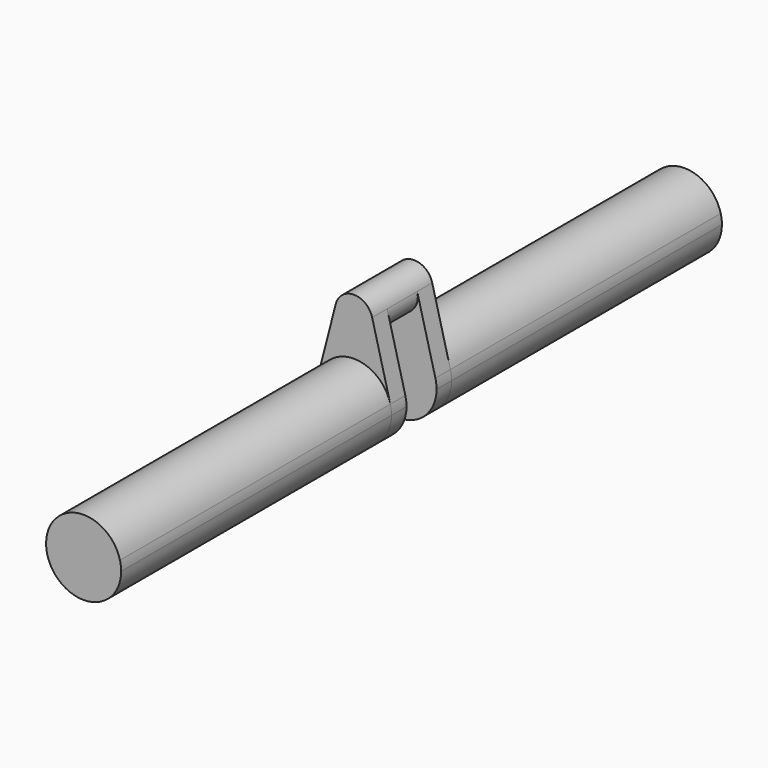
from build123d import *

# Parameters (mm, degrees)
F1_DEPTH = 5
F2_DEPTH = 50
F3_DEPTH = 2.5


with BuildPart() as f1:
    # F0 (on Front) → F1 (new body, symmetric)
    with BuildSketch(Plane.XZ):
        with BuildLine():
            ThreePointArc((2.5, 10), (2.4800742407, 10.3150107312), (2.4206145914, 10.625))
            ThreePointArc((2.4206145914, 10.625), (0, 12.5), (-2.4206145914, 10.625))
            ThreePointArc((-2.4206145914, 10.625), (-0.3150107312, 7.5199257593), (2.5, 10))
        make_face()
        with BuildLine():
            ThreePointArc((-4.8412291828, 1.25), (0, 5), (4.8412291828, 1.25))
            Line((4.8412291828, 1.25), (2.4206145914, 10.625))
            ThreePointArc((2.4206145914, 10.625), (2.4800742407, 10.3150107312), (2.5, 10))
            ThreePointArc((2.5, 10), (-0.3150107312, 7.5199257593), (-2.4206145914, 10.625))
            Line((-2.4206145914, 10.625), (-4.8412291828, 1.25))
        make_face()
        with BuildLine():
            ThreePointArc((-4.8412291828, 1.25), (-0.6300214624, -4.9601484813), (5, 0))
            ThreePointArc((5, 0), (4.9601484813, 0.6300214624), (4.8412291828, 1.25))
            ThreePointArc((4.8412291828, 1.25), (0, 5), (-4.8412291828, 1.25))
        make_face()
    extrude(amount=F1_DEPTH, both=True)

    # F0 (on Front) → F2 (join, symmetric)
    with BuildSketch(Plane.XZ):
        with BuildLine():
            ThreePointArc((-4.8412291828, 1.25), (-0.6300214624, -4.9601484813), (5, 0))
            ThreePointArc((5, 0), (4.9601484813, 0.6300214624), (4.8412291828, 1.25))
            ThreePointArc((4.8412291828, 1.25), (0, 5), (-4.8412291828, 1.25))
        make_face()
    extrude(amount=F2_DEPTH, both=True)

    # F0 (on Front) → F3 (cut, symmetric)
    with BuildSketch(Plane.XZ):
        with BuildLine():
            ThreePointArc((-4.8412291828, 1.25), (0, 5), (4.8412291828, 1.25))
            Line((4.8412291828, 1.25), (2.4206145914, 10.625))
            ThreePointArc((2.4206145914, 10.625), (2.4800742407, 10.3150107312), (2.5, 10))
            ThreePointArc((2.5, 10), (-0.3150107312, 7.5199257593), (-2.4206145914, 10.625))
            Line((-2.4206145914, 10.625), (-4.8412291828, 1.25))
        make_face()
        with BuildLine():
            ThreePointArc((-4.8412291828, 1.25), (-0.6300214624, -4.9601484813), (5, 0))
            ThreePointArc((5, 0), (4.9601484813, 0.6300214624), (4.8412291828, 1.25))
            ThreePointArc((4.8412291828, 1.25), (0, 5), (-4.8412291828, 1.25))
        make_face()
    extrude(amount=F3_DEPTH, both=True, mode=Mode.SUBTRACT)


solid = f1.part
